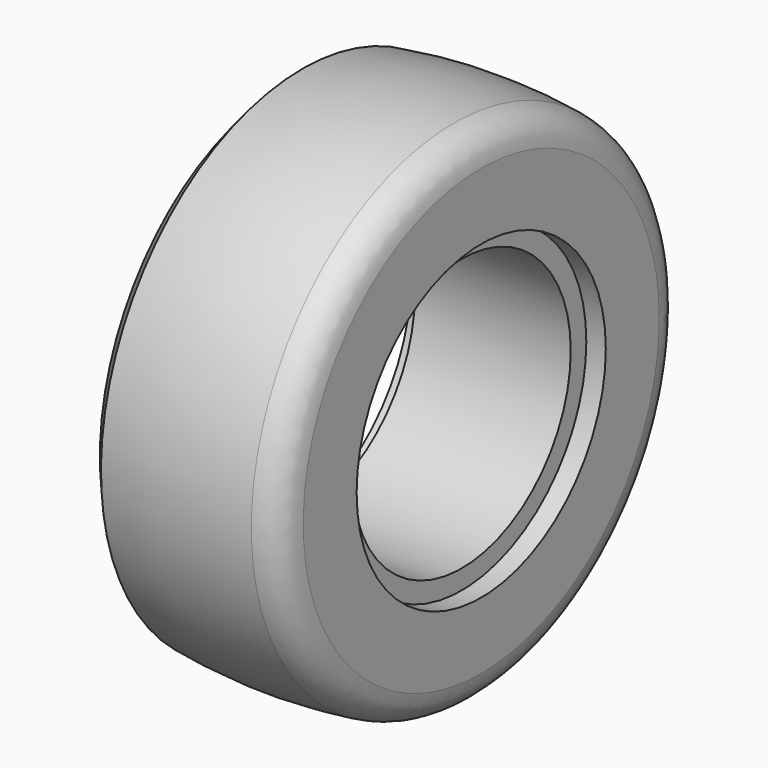
from build123d import *

# Parameters (mm, degrees)
F2_R     = 17.5
F3_DEPTH = 20
F4_R     = 4


# Not quite as in the source:
# - a fillet or chamfer that OpenCascade refuses, or shapes differently, is made with other operations: its cross-section is extruded or revolved along the edge and cut away or added


with BuildPart() as f1:
    # F0 (on Top) → F1 (revolve)
    with BuildSketch(Plane.XY):
        with BuildLine():
            Line((-10, 20), (-10, 0))
            Line((-10, 0), (10, 0))
            Line((10, 0), (10, 20))
            Line((10, 20), (12.5, 20))
            Line((12.5, 20), (12.5, 32))
            ThreePointArc((12.5, 32), (0, 33.1251134302), (-12.5, 32))
            Line((-12.5, 32), (-12.5, 20))
            Line((-12.5, 20), (-10, 20))
        make_face()
    revolve(axis=Axis((0, 0, 0), (1, 0, 0)))

    # F2 (on face) → F3 (cut, through all)
    with BuildSketch(Plane.YZ.offset(10)):
        Circle(F2_R)
    extrude(amount=-F3_DEPTH, mode=Mode.SUBTRACT)

    # F4
    f4_edges = [f1.edges().sort_by_distance(p)[0] for p in [
        (12.5, -32, 0),
    ]]
    fillet(f4_edges, radius=F4_R)

    # F5: chamfer of 2 on 1 edges, made by hand

    # F5_s1 → F5_t2 (revolve, cut)
    with BuildSketch(Plane.XY):
        with BuildLine():
            Line((-10.4102425429, 32.3994742196), (-12.5521700899, 29.9094378777))
            Line((-12.5521700899, 29.9094378777), (-12.5921700899, 29.9094378777))
            ThreePointArc((-12.5921700899, 29.9094378777), (-12.54, 30.9547189388), (-12.54, 32))
            Line((-12.54, 32), (-12.5071428571, 32.039357078))
            ThreePointArc((-12.5071428571, 32.039357078), (-11.4587168856, 32.2214187391), (-10.4162210644, 32.4390249122))
            Line((-10.4162210644, 32.4390249122), (-10.4102425429, 32.3994742196))
        make_face()
    revolve(axis=Axis((-12.5, 0, 0), (1, 0, 0)), mode=Mode.SUBTRACT)


solid = f1.part
